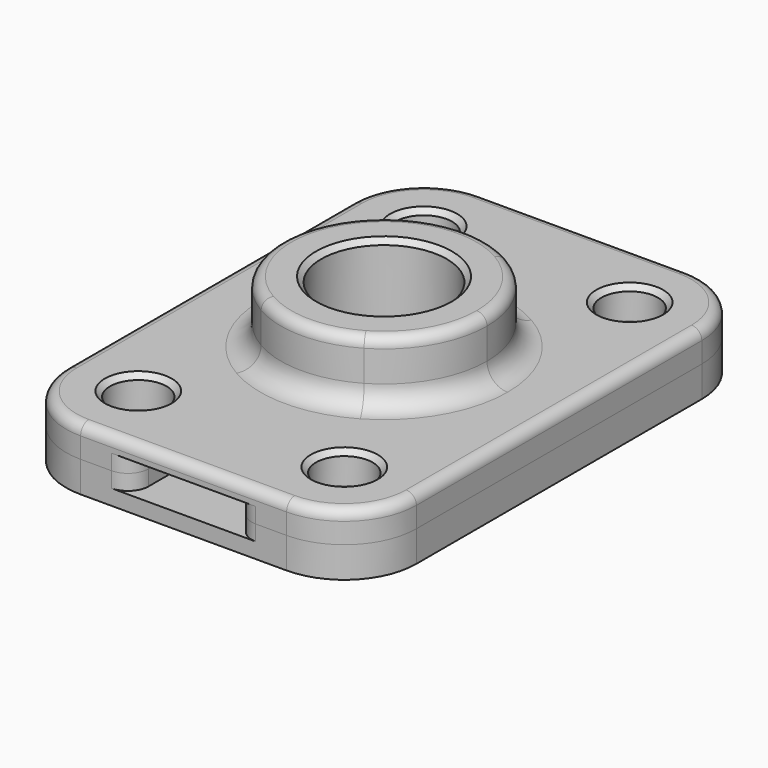
from build123d import *

# Parameters (mm, degrees)
F0_R          = 2.75
F0_R_2        = 9.25
F0_R_3        = 6.1
F1_DEPTH      = 3
F2_DEPTH      = 9
F3_DEPTH      = 1.5
F4_SIZE       = 0.5
F0_R_4        = 5
F5_DEPTH      = 3
F6_DEPTH      = 1.5
F7_R          = 2
F7_2_R        = 2
F8_F1_R       = 1
F8_F2_R       = 1
F8_F3_R       = 1
F8_F4_R       = 1
F8_F5_R       = 1
F8_F6_R       = 1
F8_2_T4_ANGLE = 148.66835306
F8_2_T9_ANGLE = 148.66835306


# Not quite as in the source:
# - a fillet or chamfer that OpenCascade refuses, or shapes differently, is made with other operations: its cross-section is extruded or revolved along the edge and cut away or added
# - a feature names something its author has since deleted; it is built from what else it names


with BuildPart() as f1:
    # F0 (on Top) → F1 (new body)
    with BuildSketch(Plane.XY):
        with BuildLine():
            ThreePointArc((-15, 8.6602540378), (-20, 17.3205080757), (-15, 25.9807621135))
            Line((-15, 25.9807621135), (-15, 41.6410161514))
            Line((-15, 41.6410161514), (-20, 41.6410161514))
            ThreePointArc((-20, 41.6410161514), (-24.9497474683, 39.5907636197), (-27, 34.6410161514))
            Line((-27, 34.6410161514), (-27, 17.3205080757))
            Line((-27, 17.3205080757), (-27, 0))
            ThreePointArc((-27, 0), (-24.9497474683, -4.9497474683), (-20, -7))
            Line((-20, -7), (-15, -7))
            Line((-15, -7), (-15, 8.6602540378))
        make_face()
        with Locations((-20, 0)):
            Circle(F0_R, mode=Mode.SUBTRACT)
        with Locations((-20, 34.6410161514)):
            Circle(F0_R, mode=Mode.SUBTRACT)
        with BuildLine():
            ThreePointArc((-5, 8.6602540378), (-1.3397459622, 12.3205080757), (0, 17.3205080757))
            ThreePointArc((0, 17.3205080757), (-1.3397459622, 22.3205080757), (-5, 25.9807621135))
            ThreePointArc((-5, 25.9807621135), (-10, 27.3205080757), (-15, 25.9807621135))
            ThreePointArc((-15, 25.9807621135), (-20, 17.3205080757), (-15, 8.6602540378))
            ThreePointArc((-15, 8.6602540378), (-10, 7.3205080757), (-5, 8.6602540378))
        make_face()
        with Locations((-10, 17.3205080757)):
            Circle(F0_R_2, mode=Mode.SUBTRACT)
        with BuildLine():
            Line((-5, -7), (-5, 8.6602540378))
            ThreePointArc((-5, 8.6602540378), (-10, 7.3205080757), (-15, 8.6602540378))
            Line((-15, 8.6602540378), (-15, -7))
            Line((-15, -7), (-10, -7))
            Line((-10, -7), (-5, -7))
        make_face()
        with BuildLine():
            ThreePointArc((-15, 25.9807621135), (-10, 27.3205080757), (-5, 25.9807621135))
            Line((-5, 25.9807621135), (-5, 41.6410161514))
            Line((-5, 41.6410161514), (-10, 41.6410161514))
            Line((-10, 41.6410161514), (-15, 41.6410161514))
            Line((-15, 41.6410161514), (-15, 25.9807621135))
        make_face()
        with BuildLine():
            ThreePointArc((-5, 25.9807621135), (-1.3397459622, 22.3205080757), (0, 17.3205080757))
            ThreePointArc((0, 17.3205080757), (-1.3397459622, 12.3205080757), (-5, 8.6602540378))
            Line((-5, 8.6602540378), (-5, -7))
            Line((-5, -7), (0, -7))
            ThreePointArc((0, -7), (4.9497474683, -4.9497474683), (7, 0))
            Line((7, 0), (7, 17.3205080757))
            Line((7, 17.3205080757), (7, 34.6410161514))
            ThreePointArc((7, 34.6410161514), (4.9497474683, 39.5907636197), (0, 41.6410161514))
            Line((0, 41.6410161514), (-5, 41.6410161514))
            Line((-5, 41.6410161514), (-5, 25.9807621135))
        make_face()
        Circle(F0_R, mode=Mode.SUBTRACT)
        with Locations((0, 34.6410161514)):
            Circle(F0_R, mode=Mode.SUBTRACT)
        with Locations((-10, 17.3205080757)):
            Circle(F0_R_2)
        with Locations((-10, 17.3205080757)):
            Circle(F0_R_3, mode=Mode.SUBTRACT)
    extrude(amount=F1_DEPTH)

    # F0 (on Top) → F2 (join)
    with BuildSketch(Plane.XY):
        with BuildLine():
            ThreePointArc((-5, 8.6602540378), (-1.3397459622, 12.3205080757), (0, 17.3205080757))
            ThreePointArc((0, 17.3205080757), (-1.3397459622, 22.3205080757), (-5, 25.9807621135))
            ThreePointArc((-5, 25.9807621135), (-10, 27.3205080757), (-15, 25.9807621135))
            ThreePointArc((-15, 25.9807621135), (-20, 17.3205080757), (-15, 8.6602540378))
            ThreePointArc((-15, 8.6602540378), (-10, 7.3205080757), (-5, 8.6602540378))
        make_face()
        with Locations((-10, 17.3205080757)):
            Circle(F0_R_2, mode=Mode.SUBTRACT)
        with Locations((-10, 17.3205080757)):
            Circle(F0_R_2)
        with Locations((-10, 17.3205080757)):
            Circle(F0_R_3, mode=Mode.SUBTRACT)
    extrude(amount=F2_DEPTH)

    # F0 (on Top) → F3 (cut)
    with BuildSketch(Plane.XY):
        with BuildLine():
            ThreePointArc((-5, 8.6602540378), (-1.3397459622, 12.3205080757), (0, 17.3205080757))
            ThreePointArc((0, 17.3205080757), (-1.3397459622, 22.3205080757), (-5, 25.9807621135))
            ThreePointArc((-5, 25.9807621135), (-10, 27.3205080757), (-15, 25.9807621135))
            ThreePointArc((-15, 25.9807621135), (-20, 17.3205080757), (-15, 8.6602540378))
            ThreePointArc((-15, 8.6602540378), (-10, 7.3205080757), (-5, 8.6602540378))
        make_face()
        with Locations((-10, 17.3205080757)):
            Circle(F0_R_2, mode=Mode.SUBTRACT)
        with Locations((-10, 17.3205080757)):
            Circle(F0_R_2)
        with Locations((-10, 17.3205080757)):
            Circle(F0_R_3, mode=Mode.SUBTRACT)
        with BuildLine():
            Line((-5, -7), (-5, 8.6602540378))
            ThreePointArc((-5, 8.6602540378), (-10, 7.3205080757), (-15, 8.6602540378))
            Line((-15, 8.6602540378), (-15, -7))
            Line((-15, -7), (-10, -7))
            Line((-10, -7), (-5, -7))
        make_face()
        with BuildLine():
            ThreePointArc((-15, 25.9807621135), (-10, 27.3205080757), (-5, 25.9807621135))
            Line((-5, 25.9807621135), (-5, 41.6410161514))
            Line((-5, 41.6410161514), (-10, 41.6410161514))
            Line((-10, 41.6410161514), (-15, 41.6410161514))
            Line((-15, 41.6410161514), (-15, 25.9807621135))
        make_face()
    extrude(amount=F3_DEPTH, mode=Mode.SUBTRACT)

    # F4
    f4_edges = [f1.edges().sort_by_distance(p)[0] for p in [
        (-16.1, 17.320508, 9),
        (-22.75, 0, 3),
        (-22.75, 34.641016, 3),
        (-2.75, 34.641016, 3),
        (-2.75, 0, 3),
    ]]
    chamfer(f4_edges, length=F4_SIZE)

    # F7
    f7_edges = [f1.edges().sort_by_distance(p)[0] for p in [
        (-15, 25.980762, 3),
        (-5, -7, 0.75),
        (-15, -7, 0.75),
        (-15, 41.641016, 0.75),
        (-5, 41.641016, 0.75),
    ]]
    fillet(f7_edges, radius=F7_R)

    # F8: fillet of radius 1 on 13 edges, made by hand

    # F8_f1
    f8_f1_edges = [f1.edges().sort_by_distance(p)[0] for p in [
        (-24.9497474683, 39.5907636197, 3),
        (-10, 41.6410161514, 3),
        (-27, 17.3205080757, 3),
        (4.9497474683, 39.5907636197, 3),
        (-24.9497474683, -4.9497474683, 3),
        (7, 17.3205080757, 3),
        (-10, -7, 3),
        (4.9497474683, -4.9497474683, 3),
    ]]
    fillet(f8_f1_edges, radius=F8_F1_R)

    # F8_f2
    f8_f2_edges = [f1.edges().sort_by_distance(p)[0] for p in [
        (-15, 25.9807621135, 9),
    ]]
    fillet(f8_f2_edges, radius=F8_F2_R)

    # F8_f3
    f8_f3_edges = [f1.edges().sort_by_distance(p)[0] for p in [
        (-15, 25.9807621135, 0.75),
    ]]
    fillet(f8_f3_edges, radius=F8_F3_R)

    # F8_f4
    f8_f4_edges = [f1.edges().sort_by_distance(p)[0] for p in [
        (-15, 8.6602540378, 0.75),
    ]]
    fillet(f8_f4_edges, radius=F8_F4_R)

    # F8_f5
    f8_f5_edges = [f1.edges().sort_by_distance(p)[0] for p in [
        (-5, 25.9807621135, 0.75),
    ]]
    fillet(f8_f5_edges, radius=F8_F5_R)

    # F8_f6
    f8_f6_edges = [f1.edges().sort_by_distance(p)[0] for p in [
        (-5, 8.6602540378, 0.75),
    ]]
    fillet(f8_f6_edges, radius=F8_F6_R)


with BuildPart() as f5:
    # F0 (on Top) → F5 (new body)
    with BuildSketch(Plane.XY):
        with BuildLine():
            ThreePointArc((-15, 8.6602540378), (-20, 17.3205080757), (-15, 25.9807621135))
            Line((-15, 25.9807621135), (-15, 41.6410161514))
            Line((-15, 41.6410161514), (-20, 41.6410161514))
            ThreePointArc((-20, 41.6410161514), (-24.9497474683, 39.5907636197), (-27, 34.6410161514))
            Line((-27, 34.6410161514), (-27, 17.3205080757))
            Line((-27, 17.3205080757), (-27, 0))
            ThreePointArc((-27, 0), (-24.9497474683, -4.9497474683), (-20, -7))
            Line((-20, -7), (-15, -7))
            Line((-15, -7), (-15, 8.6602540378))
        make_face()
        with Locations((-20, 0)):
            Circle(F0_R, mode=Mode.SUBTRACT)
        with Locations((-20, 34.6410161514)):
            Circle(F0_R, mode=Mode.SUBTRACT)
        with BuildLine():
            ThreePointArc((-5, 25.9807621135), (-1.3397459622, 22.3205080757), (0, 17.3205080757))
            ThreePointArc((0, 17.3205080757), (-1.3397459622, 12.3205080757), (-5, 8.6602540378))
            Line((-5, 8.6602540378), (-5, -7))
            Line((-5, -7), (0, -7))
            ThreePointArc((0, -7), (4.9497474683, -4.9497474683), (7, 0))
            Line((7, 0), (7, 17.3205080757))
            Line((7, 17.3205080757), (7, 34.6410161514))
            ThreePointArc((7, 34.6410161514), (4.9497474683, 39.5907636197), (0, 41.6410161514))
            Line((0, 41.6410161514), (-5, 41.6410161514))
            Line((-5, 41.6410161514), (-5, 25.9807621135))
        make_face()
        Circle(F0_R, mode=Mode.SUBTRACT)
        with Locations((0, 34.6410161514)):
            Circle(F0_R, mode=Mode.SUBTRACT)
        with BuildLine():
            ThreePointArc((-5, 8.6602540378), (-1.3397459622, 12.3205080757), (0, 17.3205080757))
            ThreePointArc((0, 17.3205080757), (-1.3397459622, 22.3205080757), (-5, 25.9807621135))
            ThreePointArc((-5, 25.9807621135), (-10, 27.3205080757), (-15, 25.9807621135))
            ThreePointArc((-15, 25.9807621135), (-20, 17.3205080757), (-15, 8.6602540378))
            ThreePointArc((-15, 8.6602540378), (-10, 7.3205080757), (-5, 8.6602540378))
        make_face()
        with Locations((-10, 17.3205080757)):
            Circle(F0_R_2, mode=Mode.SUBTRACT)
        with Locations((-10, 17.3205080757)):
            Circle(F0_R_2)
        with Locations((-10, 17.3205080757)):
            Circle(F0_R_3, mode=Mode.SUBTRACT)
        with BuildLine():
            Line((-5, -7), (-5, 8.6602540378))
            ThreePointArc((-5, 8.6602540378), (-10, 7.3205080757), (-15, 8.6602540378))
            Line((-15, 8.6602540378), (-15, -7))
            Line((-15, -7), (-10, -7))
            Line((-10, -7), (-5, -7))
        make_face()
        with BuildLine():
            ThreePointArc((-15, 25.9807621135), (-10, 27.3205080757), (-5, 25.9807621135))
            Line((-5, 25.9807621135), (-5, 41.6410161514))
            Line((-5, 41.6410161514), (-10, 41.6410161514))
            Line((-10, 41.6410161514), (-15, 41.6410161514))
            Line((-15, 41.6410161514), (-15, 25.9807621135))
        make_face()
        with Locations((-10, 17.3205080757)):
            Circle(F0_R_3)
        with Locations((-10, 17.3205080757)):
            Circle(F0_R_4, mode=Mode.SUBTRACT)
        with Locations((-10, 17.3205080757)):
            Circle(F0_R_4)
    extrude(amount=-F5_DEPTH)

    # F0 (on Top) → F6 (cut)
    with BuildSketch(Plane.XY):
        with BuildLine():
            Line((-5, -7), (-5, 8.6602540378))
            ThreePointArc((-5, 8.6602540378), (-10, 7.3205080757), (-15, 8.6602540378))
            Line((-15, 8.6602540378), (-15, -7))
            Line((-15, -7), (-10, -7))
            Line((-10, -7), (-5, -7))
        make_face()
        with BuildLine():
            ThreePointArc((-5, 8.6602540378), (-1.3397459622, 12.3205080757), (0, 17.3205080757))
            ThreePointArc((0, 17.3205080757), (-1.3397459622, 22.3205080757), (-5, 25.9807621135))
            ThreePointArc((-5, 25.9807621135), (-10, 27.3205080757), (-15, 25.9807621135))
            ThreePointArc((-15, 25.9807621135), (-20, 17.3205080757), (-15, 8.6602540378))
            ThreePointArc((-15, 8.6602540378), (-10, 7.3205080757), (-5, 8.6602540378))
        make_face()
        with Locations((-10, 17.3205080757)):
            Circle(F0_R_2, mode=Mode.SUBTRACT)
        with BuildLine():
            ThreePointArc((-15, 25.9807621135), (-10, 27.3205080757), (-5, 25.9807621135))
            Line((-5, 25.9807621135), (-5, 41.6410161514))
            Line((-5, 41.6410161514), (-10, 41.6410161514))
            Line((-10, 41.6410161514), (-15, 41.6410161514))
            Line((-15, 41.6410161514), (-15, 25.9807621135))
        make_face()
    extrude(amount=-F6_DEPTH, mode=Mode.SUBTRACT)

    # F7#2
    f7_2_edges = [f5.edges().sort_by_distance(p)[0] for p in [
        (-15, 41.641016, -0.75),
        (-5, 41.641016, -0.75),
        (-15, -7, -0.75),
        (-5, -7, -0.75),
    ]]
    fillet(f7_2_edges, radius=F7_2_R)

    # F8#2: fillet of radius 1 on 2 edges, made by hand


with BuildPart() as f8_2_tool2:
    # F8_2_s3 → F8_2_t4 (revolve)
    with BuildSketch(Plane(origin=(-4.7676046878, -1.3370452184, 0), x_dir=(0, 0, 1), z_dir=(-0.9628529864, -0.270026159, 0))):
        with BuildLine():
            ThreePointArc((-1.5, 10.377364517), (-1.2071067812, 9.6702577358), (-0.5, 9.377364517))
            Line((-0.5, 9.377364517), (-1.5, 9.377364517))
            Line((-1.5, 9.377364517), (-1.5, 10.377364517))
        make_face()
    revolve(axis=Axis((-10, 17.3205080757, -1.5), (0, 0, 1)), revolution_arc=F8_2_T4_ANGLE)

    split(bisect_by=Plane.YZ.offset(-5), keep=Keep.TOP)


with BuildPart() as f5_1:
    add(f5.part)

    # F8_2_t1: union F8_2_tool2
    add(f8_2_tool2.part)


with BuildPart() as f8_2_tool7:
    # F8_2_s8 → F8_2_t9 (revolve)
    with BuildSketch(Plane(origin=(-4.7676046878, -1.3370452184, 0), x_dir=(0, 0, 1), z_dir=(0.9628529864, 0.270026159, 0))):
        with BuildLine():
            ThreePointArc((-1.5, -28.377364517), (-1.2071067812, -29.0844712982), (-0.5, -29.377364517))
            Line((-0.5, -29.377364517), (-1.5, -29.377364517))
            Line((-1.5, -29.377364517), (-1.5, -28.377364517))
        make_face()
    revolve(axis=Axis((-10, 17.3205080757, -1.5), (0, 0, 1)), revolution_arc=F8_2_T9_ANGLE)

    split(bisect_by=Plane.YZ.offset(-15), keep=Keep.BOTTOM)


with BuildPart() as f5_2:
    add(f5_1.part)

    # F8_2_t6: union F8_2_tool7
    add(f8_2_tool7.part)


solid = Compound([f1.part, f5_2.part])
